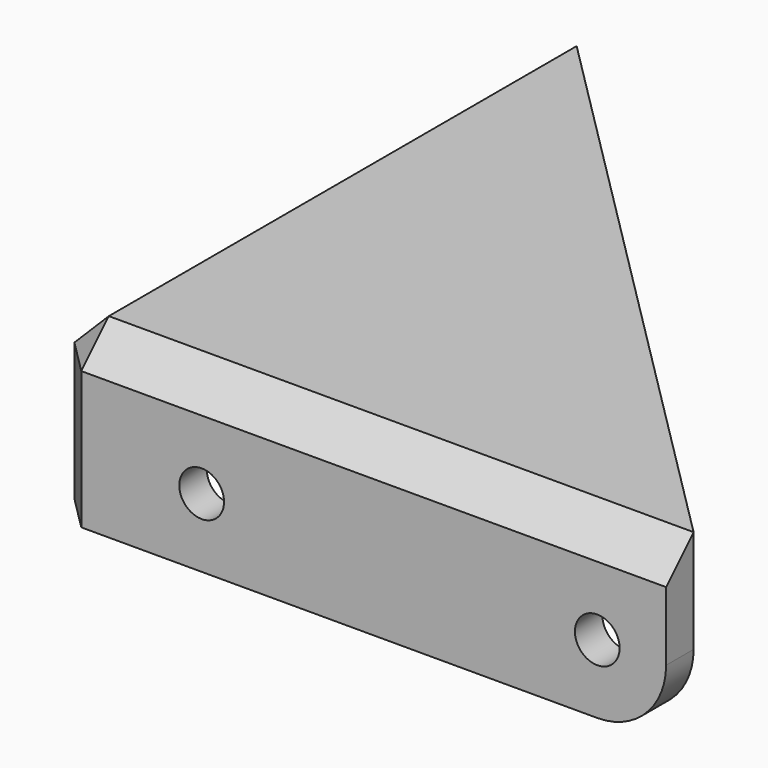
from build123d import *

# Parameters (mm, degrees)
F0_W       = 12
F0_H       = 25
F0_W_2     = 25
F0_H_2     = 12
F1_DEPTH   = 5
F2_DEPTH   = 20
F3_R       = 10
F5_R       = 3.25
F6_DEPTH   = 25
F4_R       = 3
F4_R_2     = 3.25
F7_DEPTH   = 25
F8_SIZE2   = 11.99999
F8_SIZE    = 19.99999
F8_2_SIZE2 = 11.99999
F8_2_SIZE  = 19.99999
F9_SIZE    = 5


# Not quite as in the source:
# - a fillet or chamfer is up to 0.001 mm smaller than in the source, because OpenCascade refuses the exact size


with BuildPart() as f1:
    # F0 (on Top) → F1 (new body)
    with BuildSketch(Plane.XY):
        Polygon((0, 90), (0, 0), (90, 0), (90, 5), (60, 5), (35, 5), (5, 5), (5, 35), (5, 60), (5, 90), align=None)
        Polygon((90, 5), (5, 90), (5, 60), (17, 60), (17, 35), (5, 35), (5, 5), (35, 5), (35, 17), (60, 17), (60, 5), align=None)
        with Locations((11, 47.5)):
            Rectangle(F0_W, F0_H)
        with Locations((47.5, 11)):
            Rectangle(F0_W_2, F0_H_2)
    extrude(amount=F1_DEPTH)

    # F0 (on Top) → F2 (join)
    with BuildSketch(Plane.XY):
        Polygon((0, 90), (0, 0), (90, 0), (90, 5), (60, 5), (35, 5), (5, 5), (5, 35), (5, 60), (5, 90), align=None)
        with Locations((11, 47.5)):
            Rectangle(F0_W, F0_H)
        with Locations((47.5, 11)):
            Rectangle(F0_W_2, F0_H_2)
    extrude(amount=-F2_DEPTH)

    # F3
    f3_edges = [f1.edges().sort_by_distance(p)[0] for p in [
        (5, 5, -10),
        (2.5, 90, -20),
        (90, 2.5, -20),
    ]]
    fillet(f3_edges, radius=F3_R)

    # F5 (on face) → F6 (cut)
    with BuildSketch(Plane.XZ):
        with Locations((22.5, -10)):
            Circle(F5_R)
        with Locations((80, -10)):
            Circle(F5_R)
    extrude(amount=-F6_DEPTH, mode=Mode.SUBTRACT)

    # F4 (on face) → F7 (cut)
    with BuildSketch(Plane(origin=(0, 0, 0), x_dir=(0, -1, 0), z_dir=(-1, 0, 0))):
        with Locations((-22.5, -10)):
            Circle(F4_R)
        with Locations((-80, -10)):
            Circle(F4_R_2)
    extrude(amount=-F7_DEPTH, mode=Mode.SUBTRACT)

    # F8 (size 20 and 12 in the source; OpenCascade refuses exactly that, so slightly less here)
    f8_edges = [f1.edges().sort_by_distance(p)[0] for p in [
        (17, 47.5, -20),
    ]]
    f8_side = f1.faces().sort_by_distance((17, 47.5, -10))[0]
    chamfer(f8_edges, length=F8_SIZE, length2=F8_SIZE2, reference=f8_side)

    # F8#2 (size 20 and 12 in the source; OpenCascade refuses exactly that, so slightly less here)
    f8_2_edges = [f1.edges().sort_by_distance(p)[0] for p in [
        (47.5, 17, -20),
    ]]
    f8_2_side = f1.faces().sort_by_distance((47.5, 17, -10))[0]
    chamfer(f8_2_edges, length=F8_2_SIZE, length2=F8_2_SIZE2, reference=f8_2_side)

    # F9
    f9_edges = [f1.edges().sort_by_distance(p)[0] for p in [
        (0, 0, -7.5),
        (45, 0, 5),
        (0, 45, 5),
    ]]
    chamfer(f9_edges, length=F9_SIZE)


solid = f1.part
